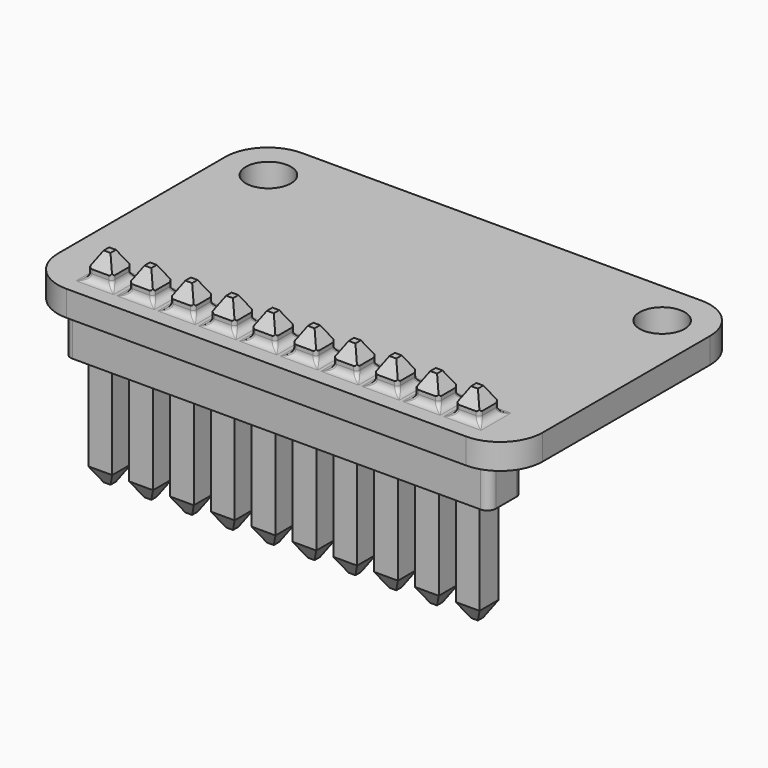
from build123d import *

# Parameters (mm, degrees)
F0_W          = 28.5
F0_H          = 17.3
F0_R          = 1.825
F1_DEPTH      = 1.5
F2_R          = 2.5
F3_R          = 1.825
F3_R_2        = 1.325
F4_DEPTH      = 1.5
F5_W          = 25
F5_H          = 2.5
F6_DEPTH      = 2.5
F7_R          = 0.5
F8_W          = 1.4
F8_H          = 1.4
F9_DEPTH      = 6.5
F9_DEPTH_BACK = 5.5
F10_R         = 0.4
F11_SIZE2     = 0.8660254038
F11_SIZE      = 0.5
F11_2_SIZE2   = 0.8660254038
F11_2_SIZE    = 0.5
F11_3_SIZE2   = 0.8660254038
F11_3_SIZE    = 0.5
F11_4_SIZE2   = 0.8660254038
F11_4_SIZE    = 0.5
F11_5_SIZE2   = 0.8660254038
F11_5_SIZE    = 0.5
F11_6_SIZE2   = 0.8660254038
F11_6_SIZE    = 0.5
F11_7_SIZE2   = 0.8660254038
F11_7_SIZE    = 0.5
F11_8_SIZE2   = 0.8660254038
F11_8_SIZE    = 0.5
F11_9_SIZE2   = 0.8660254038
F11_9_SIZE    = 0.5
F11_10_SIZE2  = 0.8660254038
F11_10_SIZE   = 0.5
F11_11_SIZE2  = 0.8660254038
F11_11_SIZE   = 0.5
F11_12_SIZE2  = 0.8660254038
F11_12_SIZE   = 0.5
F11_13_SIZE2  = 0.8660254038
F11_13_SIZE   = 0.5
F11_14_SIZE2  = 0.8660254038
F11_14_SIZE   = 0.5
F11_15_SIZE2  = 0.8660254038
F11_15_SIZE   = 0.5
F11_16_SIZE2  = 0.8660254038
F11_16_SIZE   = 0.5
F11_17_SIZE2  = 0.8660254038
F11_17_SIZE   = 0.5
F11_18_SIZE2  = 0.8660254038
F11_18_SIZE   = 0.5
F11_19_SIZE2  = 0.8660254038
F11_19_SIZE   = 0.5
F11_20_SIZE2  = 0.8660254038
F11_20_SIZE   = 0.5
F12_SIZE2     = 0.8660254038
F12_SIZE      = 0.5
F12_2_SIZE2   = 0.8660254038
F12_2_SIZE    = 0.5
F12_3_SIZE2   = 0.8660254038
F12_3_SIZE    = 0.5
F12_4_SIZE2   = 0.8660254038
F12_4_SIZE    = 0.5
F12_5_SIZE2   = 0.8660254038
F12_5_SIZE    = 0.5
F12_6_SIZE2   = 0.8660254038
F12_6_SIZE    = 0.5
F12_7_SIZE2   = 0.8660254038
F12_7_SIZE    = 0.5
F12_8_SIZE2   = 0.8660254038
F12_8_SIZE    = 0.5
F12_9_SIZE2   = 0.8660254038
F12_9_SIZE    = 0.5
F12_10_SIZE2  = 0.8660254038
F12_10_SIZE   = 0.5
F12_11_SIZE2  = 0.8660254038
F12_11_SIZE   = 0.5
F12_12_SIZE2  = 0.8660254038
F12_12_SIZE   = 0.5
F12_13_SIZE2  = 0.8660254038
F12_13_SIZE   = 0.5
F12_14_SIZE2  = 0.8660254038
F12_14_SIZE   = 0.5
F12_15_SIZE2  = 0.8660254038
F12_15_SIZE   = 0.5
F12_16_SIZE2  = 0.8660254038
F12_16_SIZE   = 0.5
F12_17_SIZE2  = 0.8660254038
F12_17_SIZE   = 0.5
F12_18_SIZE2  = 0.8660254038
F12_18_SIZE   = 0.5
F12_19_SIZE2  = 0.8660254038
F12_19_SIZE   = 0.5
F13_R         = 0.2


with BuildPart() as f1:
    # F0 (on Top) → F1 (new body)
    with BuildSketch(Plane.XY):
        Rectangle(F0_W, F0_H)
        with Locations((-11.575, 5.975)):
            Circle(F0_R, mode=Mode.SUBTRACT)
        with Locations((11.575, 5.975)):
            Circle(F0_R, mode=Mode.SUBTRACT)
    extrude(amount=F1_DEPTH)

    # F2
    f2_edges = [f1.edges().sort_by_distance(p)[0] for p in [
        (14.25, 8.65, 0.75),
        (-14.25, 8.65, 0.75),
        (-14.25, -8.65, 0.75),
        (14.25, -8.65, 0.75),
    ]]
    fillet(f2_edges, radius=F2_R)

    # F3 (on face) → F4 (join)
    with BuildSketch(Plane.XY.offset(1.5)):
        with Locations((-11.575, 5.975)):
            Circle(F3_R)
        with Locations((-11.575, 5.975)):
            Circle(F3_R_2, mode=Mode.SUBTRACT)
        with Locations((11.575, 5.975)):
            Circle(F3_R)
        with Locations((11.575, 5.975)):
            Circle(F3_R_2, mode=Mode.SUBTRACT)
    extrude(amount=-F4_DEPTH)



with BuildPart() as f6:
    # F5 (on face) → F6 (new body)
    with BuildSketch(Plane(origin=(0, 0, 0), x_dir=(1, 0, 0), z_dir=(0, 0, -1))):
        with Locations((0, 6.65)):
            Rectangle(F5_W, F5_H)
    extrude(amount=F6_DEPTH)

    # F7
    f7_edges = [f6.edges().sort_by_distance(p)[0] for p in [
        (12.5, -7.9, -1.25),
        (-12.5, -7.9, -1.25),
        (-12.5, -5.4, -1.25),
        (12.5, -5.4, -1.25),
    ]]
    fillet(f7_edges, radius=F7_R)


with BuildPart() as f1_1:
    add(f1.part)

    add(f6.part)  # F9 merges F6
    # F8 (on face) → F9 (join, two sides)
    with BuildSketch(Plane(origin=(0, 0, -2.5), x_dir=(1, 0, 0), z_dir=(0, 0, -1))) as f9_sk:
        with Locations((-10.8, 6.65)):
            Rectangle(F8_W, F8_H)
        with Locations((-8.4, 6.65)):
            Rectangle(F8_W, F8_H)
        with Locations((-6, 6.65)):
            Rectangle(F8_W, F8_H)
        with Locations((-3.6, 6.65)):
            Rectangle(F8_W, F8_H)
        with Locations((-1.2, 6.65)):
            Rectangle(F8_W, F8_H)
        with Locations((1.2, 6.65)):
            Rectangle(F8_W, F8_H)
        with Locations((3.6, 6.65)):
            Rectangle(F8_W, F8_H)
        with Locations((6, 6.65)):
            Rectangle(F8_W, F8_H)
        with Locations((8.4, 6.65)):
            Rectangle(F8_W, F8_H)
        with Locations((10.8, 6.65)):
            Rectangle(F8_W, F8_H)
    extrude(amount=F9_DEPTH)
    extrude(f9_sk.sketch, amount=-F9_DEPTH_BACK)

    # F10
    f10_edges = [f1_1.edges().sort_by_distance(p)[0] for p in [
        (11.5, -6.65, 1.5),
        (10.8, -7.35, 1.5),
        (10.8, -5.95, 1.5),
        (10.1, -6.65, 1.5),
        (8.4, -7.35, 1.5),
        (9.1, -6.65, 1.5),
        (8.4, -5.95, 1.5),
        (7.7, -6.65, 1.5),
        (6.7, -6.65, 1.5),
        (6, -7.35, 1.5),
        (6, -5.95, 1.5),
        (5.3, -6.65, 1.5),
        (4.3, -6.65, 1.5),
        (3.6, -7.35, 1.5),
        (3.6, -5.95, 1.5),
        (2.9, -6.65, 1.5),
        (1.2, -5.95, 1.5),
        (0.5, -6.65, 1.5),
        (1.9, -6.65, 1.5),
        (1.2, -7.35, 1.5),
        (-2.9, -6.65, 1.5),
        (-1.2, -7.35, 1.5),
        (-0.5, -6.65, 1.5),
        (-3.6, -7.35, 1.5),
        (-3.6, -5.95, 1.5),
        (-1.2, -5.95, 1.5),
        (-6, -5.95, 1.5),
        (-8.4, -5.95, 1.5),
        (-10.8, -5.95, 1.5),
        (-10.1, -6.65, 1.5),
        (-7.7, -6.65, 1.5),
        (-5.3, -6.65, 1.5),
        (-1.9, -6.65, 1.5),
        (-4.3, -6.65, 1.5),
        (-6, -7.35, 1.5),
        (-6.7, -6.65, 1.5),
        (-8.4, -7.35, 1.5),
        (-9.1, -6.65, 1.5),
        (-10.8, -7.35, 1.5),
        (-11.5, -6.65, 1.5),
    ]]
    fillet(f10_edges, radius=F10_R)

    # F11
    f11_edges = [f1_1.edges().sort_by_distance(p)[0] for p in [
        (11.5, -6.65, 3),
        (10.8, -7.35, 3),
        (10.1, -6.65, 3),
        (10.8, -5.95, 3),
    ]]
    f11_side = f1_1.faces().sort_by_distance((10.8, -6.65, 3))[0]
    chamfer(f11_edges, length=F11_SIZE, length2=F11_SIZE2, reference=f11_side)

    # F11#2
    f11_2_edges = [f1_1.edges().sort_by_distance(p)[0] for p in [
        (6.7, -6.65, 3),
        (6, -5.95, 3),
    ]]
    f11_2_side = f1_1.faces().sort_by_distance((6, -6.65, 3))[0]
    chamfer(f11_2_edges, length=F11_2_SIZE, length2=F11_2_SIZE2, reference=f11_2_side)

    # F11#3
    f11_3_edges = [f1_1.edges().sort_by_distance(p)[0] for p in [
        (-5.3, -6.65, 3),
        (-6, -5.95, 3),
    ]]
    f11_3_side = f1_1.faces().sort_by_distance((-6, -6.65, 3))[0]
    chamfer(f11_3_edges, length=F11_3_SIZE, length2=F11_3_SIZE2, reference=f11_3_side)

    # F11#4
    f11_4_edges = [f1_1.edges().sort_by_distance(p)[0] for p in [
        (-10.1, -6.65, 3),
        (-10.8, -5.95, 3),
    ]]
    f11_4_side = f1_1.faces().sort_by_distance((-10.8, -6.65, 3))[0]
    chamfer(f11_4_edges, length=F11_4_SIZE, length2=F11_4_SIZE2, reference=f11_4_side)

    # F11#5
    f11_5_edges = [f1_1.edges().sort_by_distance(p)[0] for p in [
        (-10.8, -7.35, -9),
        (-11.5, -6.65, -9),
    ]]
    f11_5_side = f1_1.faces().sort_by_distance((-10.8, -6.65, -9))[0]
    chamfer(f11_5_edges, length=F11_5_SIZE, length2=F11_5_SIZE2, reference=f11_5_side)

    # F11#6
    f11_6_edges = [f1_1.edges().sort_by_distance(p)[0] for p in [
        (-6, -7.35, -9),
        (-6.7, -6.65, -9),
    ]]
    f11_6_side = f1_1.faces().sort_by_distance((-6, -6.65, -9))[0]
    chamfer(f11_6_edges, length=F11_6_SIZE, length2=F11_6_SIZE2, reference=f11_6_side)

    # F11#7
    f11_7_edges = [f1_1.edges().sort_by_distance(p)[0] for p in [
        (6, -7.35, -9),
        (5.3, -6.65, -9),
    ]]
    f11_7_side = f1_1.faces().sort_by_distance((6, -6.65, -9))[0]
    chamfer(f11_7_edges, length=F11_7_SIZE, length2=F11_7_SIZE2, reference=f11_7_side)

    # F11#8
    f11_8_edges = [f1_1.edges().sort_by_distance(p)[0] for p in [
        (10.8, -7.35, -9),
        (10.1, -6.65, -9),
    ]]
    f11_8_side = f1_1.faces().sort_by_distance((10.8, -6.65, -9))[0]
    chamfer(f11_8_edges, length=F11_8_SIZE, length2=F11_8_SIZE2, reference=f11_8_side)

    # F11#9
    f11_9_edges = [f1_1.edges().sort_by_distance(p)[0] for p in [
        (4.3, -6.65, 3),
        (3.6, -5.95, 3),
    ]]
    f11_9_side = f1_1.faces().sort_by_distance((3.6, -6.65, 3))[0]
    chamfer(f11_9_edges, length=F11_9_SIZE, length2=F11_9_SIZE2, reference=f11_9_side)

    # F11#10
    f11_10_edges = [f1_1.edges().sort_by_distance(p)[0] for p in [
        (1.9, -6.65, 3),
        (1.2, -5.95, 3),
    ]]
    f11_10_side = f1_1.faces().sort_by_distance((1.2, -6.65, 3))[0]
    chamfer(f11_10_edges, length=F11_10_SIZE, length2=F11_10_SIZE2, reference=f11_10_side)

    # F11#11
    f11_11_edges = [f1_1.edges().sort_by_distance(p)[0] for p in [
        (-2.9, -6.65, 3),
        (-3.6, -5.95, 3),
    ]]
    f11_11_side = f1_1.faces().sort_by_distance((-3.6, -6.65, 3))[0]
    chamfer(f11_11_edges, length=F11_11_SIZE, length2=F11_11_SIZE2, reference=f11_11_side)

    # F11#12
    f11_12_edges = [f1_1.edges().sort_by_distance(p)[0] for p in [
        (-0.5, -6.65, 3),
        (-1.2, -5.95, 3),
    ]]
    f11_12_side = f1_1.faces().sort_by_distance((-1.2, -6.65, 3))[0]
    chamfer(f11_12_edges, length=F11_12_SIZE, length2=F11_12_SIZE2, reference=f11_12_side)

    # F11#13
    f11_13_edges = [f1_1.edges().sort_by_distance(p)[0] for p in [
        (-3.6, -7.35, -9),
        (-4.3, -6.65, -9),
    ]]
    f11_13_side = f1_1.faces().sort_by_distance((-3.6, -6.65, -9))[0]
    chamfer(f11_13_edges, length=F11_13_SIZE, length2=F11_13_SIZE2, reference=f11_13_side)

    # F11#14
    f11_14_edges = [f1_1.edges().sort_by_distance(p)[0] for p in [
        (-1.2, -7.35, -9),
        (-1.9, -6.65, -9),
    ]]
    f11_14_side = f1_1.faces().sort_by_distance((-1.2, -6.65, -9))[0]
    chamfer(f11_14_edges, length=F11_14_SIZE, length2=F11_14_SIZE2, reference=f11_14_side)

    # F11#15
    f11_15_edges = [f1_1.edges().sort_by_distance(p)[0] for p in [
        (1.2, -7.35, -9),
        (0.5, -6.65, -9),
    ]]
    f11_15_side = f1_1.faces().sort_by_distance((1.2, -6.65, -9))[0]
    chamfer(f11_15_edges, length=F11_15_SIZE, length2=F11_15_SIZE2, reference=f11_15_side)

    # F11#16
    f11_16_edges = [f1_1.edges().sort_by_distance(p)[0] for p in [
        (3.6, -7.35, -9),
        (2.9, -6.65, -9),
    ]]
    f11_16_side = f1_1.faces().sort_by_distance((3.6, -6.65, -9))[0]
    chamfer(f11_16_edges, length=F11_16_SIZE, length2=F11_16_SIZE2, reference=f11_16_side)

    # F11#17
    f11_17_edges = [f1_1.edges().sort_by_distance(p)[0] for p in [
        (9.1, -6.65, 3),
        (8.4, -5.95, 3),
    ]]
    f11_17_side = f1_1.faces().sort_by_distance((8.4, -6.65, 3))[0]
    chamfer(f11_17_edges, length=F11_17_SIZE, length2=F11_17_SIZE2, reference=f11_17_side)

    # F11#18
    f11_18_edges = [f1_1.edges().sort_by_distance(p)[0] for p in [
        (-7.7, -6.65, 3),
        (-8.4, -5.95, 3),
    ]]
    f11_18_side = f1_1.faces().sort_by_distance((-8.4, -6.65, 3))[0]
    chamfer(f11_18_edges, length=F11_18_SIZE, length2=F11_18_SIZE2, reference=f11_18_side)

    # F11#19
    f11_19_edges = [f1_1.edges().sort_by_distance(p)[0] for p in [
        (-8.4, -7.35, -9),
        (-9.1, -6.65, -9),
    ]]
    f11_19_side = f1_1.faces().sort_by_distance((-8.4, -6.65, -9))[0]
    chamfer(f11_19_edges, length=F11_19_SIZE, length2=F11_19_SIZE2, reference=f11_19_side)

    # F11#20
    f11_20_edges = [f1_1.edges().sort_by_distance(p)[0] for p in [
        (8.4, -7.35, -9),
        (7.7, -6.65, -9),
    ]]
    f11_20_side = f1_1.faces().sort_by_distance((8.4, -6.65, -9))[0]
    chamfer(f11_20_edges, length=F11_20_SIZE, length2=F11_20_SIZE2, reference=f11_20_side)

    # F12
    f12_edges = [f1_1.edges().sort_by_distance(p)[0] for p in [
        (-10.55, -5.95, -9),
        (-10.1, -6.4, -9),
    ]]
    f12_side = f1_1.faces().sort_by_distance((-10.55, -6.4, -9))[0]
    chamfer(f12_edges, length=F12_SIZE, length2=F12_SIZE2, reference=f12_side)

    # F12#2
    f12_2_edges = [f1_1.edges().sort_by_distance(p)[0] for p in [
        (-8.15, -5.95, -9),
        (-7.7, -6.4, -9),
    ]]
    f12_2_side = f1_1.faces().sort_by_distance((-8.15, -6.4, -9))[0]
    chamfer(f12_2_edges, length=F12_2_SIZE, length2=F12_2_SIZE2, reference=f12_2_side)

    # F12#3
    f12_3_edges = [f1_1.edges().sort_by_distance(p)[0] for p in [
        (-5.75, -5.95, -9),
        (-5.3, -6.4, -9),
    ]]
    f12_3_side = f1_1.faces().sort_by_distance((-5.75, -6.4, -9))[0]
    chamfer(f12_3_edges, length=F12_3_SIZE, length2=F12_3_SIZE2, reference=f12_3_side)

    # F12#4
    f12_4_edges = [f1_1.edges().sort_by_distance(p)[0] for p in [
        (-3.35, -5.95, -9),
        (-2.9, -6.4, -9),
    ]]
    f12_4_side = f1_1.faces().sort_by_distance((-3.35, -6.4, -9))[0]
    chamfer(f12_4_edges, length=F12_4_SIZE, length2=F12_4_SIZE2, reference=f12_4_side)

    # F12#5
    f12_5_edges = [f1_1.edges().sort_by_distance(p)[0] for p in [
        (-0.95, -5.95, -9),
        (-0.5, -6.4, -9),
    ]]
    f12_5_side = f1_1.faces().sort_by_distance((-0.95, -6.4, -9))[0]
    chamfer(f12_5_edges, length=F12_5_SIZE, length2=F12_5_SIZE2, reference=f12_5_side)

    # F12#6
    f12_6_edges = [f1_1.edges().sort_by_distance(p)[0] for p in [
        (1.45, -5.95, -9),
        (1.9, -6.4, -9),
    ]]
    f12_6_side = f1_1.faces().sort_by_distance((1.45, -6.4, -9))[0]
    chamfer(f12_6_edges, length=F12_6_SIZE, length2=F12_6_SIZE2, reference=f12_6_side)

    # F12#7
    f12_7_edges = [f1_1.edges().sort_by_distance(p)[0] for p in [
        (3.85, -5.95, -9),
        (4.3, -6.4, -9),
    ]]
    f12_7_side = f1_1.faces().sort_by_distance((3.85, -6.4, -9))[0]
    chamfer(f12_7_edges, length=F12_7_SIZE, length2=F12_7_SIZE2, reference=f12_7_side)

    # F12#8
    f12_8_edges = [f1_1.edges().sort_by_distance(p)[0] for p in [
        (6.25, -5.95, -9),
        (6.7, -6.4, -9),
    ]]
    f12_8_side = f1_1.faces().sort_by_distance((6.25, -6.4, -9))[0]
    chamfer(f12_8_edges, length=F12_8_SIZE, length2=F12_8_SIZE2, reference=f12_8_side)

    # F12#9
    f12_9_edges = [f1_1.edges().sort_by_distance(p)[0] for p in [
        (8.65, -5.95, -9),
        (9.1, -6.4, -9),
    ]]
    f12_9_side = f1_1.faces().sort_by_distance((8.65, -6.4, -9))[0]
    chamfer(f12_9_edges, length=F12_9_SIZE, length2=F12_9_SIZE2, reference=f12_9_side)

    # F12#10
    f12_10_edges = [f1_1.edges().sort_by_distance(p)[0] for p in [
        (11.05, -5.95, -9),
        (11.5, -6.4, -9),
    ]]
    f12_10_side = f1_1.faces().sort_by_distance((11.05, -6.4, -9))[0]
    chamfer(f12_10_edges, length=F12_10_SIZE, length2=F12_10_SIZE2, reference=f12_10_side)

    # F12#11
    f12_11_edges = [f1_1.edges().sort_by_distance(p)[0] for p in [
        (8.15, -7.35, 3),
        (7.7, -6.9, 3),
    ]]
    f12_11_side = f1_1.faces().sort_by_distance((8.15, -6.9, 3))[0]
    chamfer(f12_11_edges, length=F12_11_SIZE, length2=F12_11_SIZE2, reference=f12_11_side)

    # F12#12
    f12_12_edges = [f1_1.edges().sort_by_distance(p)[0] for p in [
        (5.75, -7.35, 3),
        (5.3, -6.9, 3),
    ]]
    f12_12_side = f1_1.faces().sort_by_distance((5.75, -6.9, 3))[0]
    chamfer(f12_12_edges, length=F12_12_SIZE, length2=F12_12_SIZE2, reference=f12_12_side)

    # F12#13
    f12_13_edges = [f1_1.edges().sort_by_distance(p)[0] for p in [
        (3.35, -7.35, 3),
        (2.9, -6.9, 3),
    ]]
    f12_13_side = f1_1.faces().sort_by_distance((3.35, -6.9, 3))[0]
    chamfer(f12_13_edges, length=F12_13_SIZE, length2=F12_13_SIZE2, reference=f12_13_side)

    # F12#14
    f12_14_edges = [f1_1.edges().sort_by_distance(p)[0] for p in [
        (0.95, -7.35, 3),
        (0.5, -6.9, 3),
    ]]
    f12_14_side = f1_1.faces().sort_by_distance((0.95, -6.9, 3))[0]
    chamfer(f12_14_edges, length=F12_14_SIZE, length2=F12_14_SIZE2, reference=f12_14_side)

    # F12#15
    f12_15_edges = [f1_1.edges().sort_by_distance(p)[0] for p in [
        (-1.45, -7.35, 3),
        (-1.9, -6.9, 3),
    ]]
    f12_15_side = f1_1.faces().sort_by_distance((-1.45, -6.9, 3))[0]
    chamfer(f12_15_edges, length=F12_15_SIZE, length2=F12_15_SIZE2, reference=f12_15_side)

    # F12#16
    f12_16_edges = [f1_1.edges().sort_by_distance(p)[0] for p in [
        (-3.85, -7.35, 3),
        (-4.3, -6.9, 3),
    ]]
    f12_16_side = f1_1.faces().sort_by_distance((-3.85, -6.9, 3))[0]
    chamfer(f12_16_edges, length=F12_16_SIZE, length2=F12_16_SIZE2, reference=f12_16_side)

    # F12#17
    f12_17_edges = [f1_1.edges().sort_by_distance(p)[0] for p in [
        (-6.25, -7.35, 3),
        (-6.7, -6.9, 3),
    ]]
    f12_17_side = f1_1.faces().sort_by_distance((-6.25, -6.9, 3))[0]
    chamfer(f12_17_edges, length=F12_17_SIZE, length2=F12_17_SIZE2, reference=f12_17_side)

    # F12#18
    f12_18_edges = [f1_1.edges().sort_by_distance(p)[0] for p in [
        (-8.65, -7.35, 3),
        (-9.1, -6.9, 3),
    ]]
    f12_18_side = f1_1.faces().sort_by_distance((-8.65, -6.9, 3))[0]
    chamfer(f12_18_edges, length=F12_18_SIZE, length2=F12_18_SIZE2, reference=f12_18_side)

    # F12#19
    f12_19_edges = [f1_1.edges().sort_by_distance(p)[0] for p in [
        (-11.05, -7.35, 3),
        (-11.5, -6.9, 3),
    ]]
    f12_19_side = f1_1.faces().sort_by_distance((-11.05, -6.9, 3))[0]
    chamfer(f12_19_edges, length=F12_19_SIZE, length2=F12_19_SIZE2, reference=f12_19_side)

    # F13
    f13_edges = [f1_1.edges().sort_by_distance(p)[0] for p in [
        (11.64158, -7.49158, 1.594682),
        (11.64158, -5.80842, 1.594682),
        (9.95842, -5.80842, 1.594682),
        (9.95842, -7.49158, 1.594682),
        (9.24158, -7.49158, 1.594682),
        (7.55842, -7.49158, 1.594682),
        (7.55842, -5.80842, 1.594682),
        (9.24158, -5.80842, 1.594682),
        (6.84158, -5.80842, 1.594682),
        (6.84158, -7.49158, 1.594682),
        (5.15842, -7.49158, 1.594682),
        (5.15842, -5.80842, 1.594682),
        (4.44158, -5.80842, 1.594682),
        (4.44158, -7.49158, 1.594682),
        (2.75842, -5.80842, 1.594682),
        (2.75842, -7.49158, 1.594682),
        (2.04158, -7.49158, 1.594682),
        (2.04158, -5.80842, 1.594682),
        (0.35842, -5.80842, 1.594682),
        (0.35842, -7.49158, 1.594682),
        (-0.35842, -7.49158, 1.594682),
        (-0.35842, -5.80842, 1.594682),
        (-2.04158, -5.80842, 1.594682),
        (-2.04158, -7.49158, 1.594682),
        (-2.75842, -7.49158, 1.594682),
        (-4.44158, -7.49158, 1.594682),
        (-4.44158, -5.80842, 1.594682),
        (-2.75842, -5.80842, 1.594682),
        (-6.84158, -5.80842, 1.594682),
        (-5.15842, -5.80842, 1.594682),
        (-5.15842, -7.49158, 1.594682),
        (-6.84158, -7.49158, 1.594682),
        (-9.24158, -7.49158, 1.594682),
        (-9.24158, -5.80842, 1.594682),
        (-7.55842, -5.80842, 1.594682),
        (-7.55842, -7.49158, 1.594682),
        (-9.95842, -7.49158, 1.594682),
        (-9.95842, -5.80842, 1.594682),
        (-11.64158, -5.80842, 1.594682),
        (-11.64158, -7.49158, 1.594682),
    ]]
    fillet(f13_edges, radius=F13_R)


solid = f1_1.part
